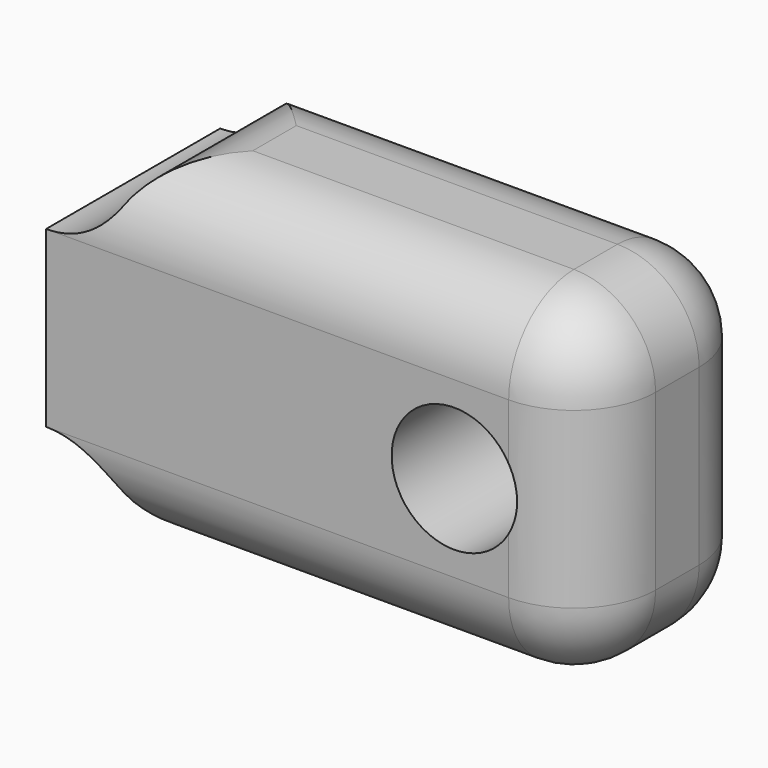
from build123d import *

# Parameters (mm, degrees)
F0_R         = 1.15
F1_DEPTH     = 4
F2_R         = 1.5
F3_DEPTH     = 5
F4_T1_DEPTH  = 9.4903810568
F4_T3_DEPTH  = 1
F4_T5_DEPTH  = 10.75
F4_T7_DEPTH  = 3.2
F4_S11_W     = 1.5
F4_S11_H     = 1.5
F4_T12_DEPTH = 1.5
F4_S17_W     = 1.5
F4_S17_H     = 1.5
F4_T18_DEPTH = 1.5
F4_S23_W     = 1.5
F4_S23_H     = 1.5
F4_T24_DEPTH = 1.5
F4_S29_W     = 1.5
F4_S29_H     = 1.5
F4_T30_DEPTH = 1.5


# Not quite as in the source:
# - a fillet or chamfer that OpenCascade refuses, or shapes differently, is made with other operations: its cross-section is extruded or revolved along the edge and cut away or added


with BuildPart() as f1:
    # F0 (on Front) → F1 (new body)
    with BuildSketch(Plane.XZ):
        with BuildLine():
            Line((5, 3.1), (-3.5, 3.1))
            ThreePointArc((-3.5, 3.1), (-3.9393398282, 2.0393398282), (-5, 1.6))
            Line((-5, 1.6), (-5, -1.6))
            ThreePointArc((-5, -1.6), (-3.9393398282, -2.0393398282), (-3.5, -3.1))
            Line((-3.5, -3.1), (5, -3.1))
            Line((5, -3.1), (5, 3.1))
        make_face()
        with Locations((2.5, 0)):
            Circle(F0_R, mode=Mode.SUBTRACT)
    extrude(amount=F1_DEPTH)

    # F2 (on face) → F3 (cut)
    with BuildSketch(Plane(origin=(-5, 0, 0), x_dir=(0, -1, 0), z_dir=(-1, 0, 0))):
        with Locations((1.9687709864, 0)):
            Circle(F2_R)
    extrude(amount=-F3_DEPTH, mode=Mode.SUBTRACT)

    # F4: fillet of radius 1.5 on 10 edges, made by hand

    # F4_s2 → F4_t1 (cut)
    with BuildSketch(Plane.XZ.offset(-2.7451905284)):
        with BuildLine():
            ThreePointArc((-2.4019237886, 3.1), (-3.1519237886, 2.8990381057), (-3.7009618943, 2.35))
            ThreePointArc((-3.7009618943, 2.35), (-3.5511112606, 2.7117714323), (-3.5, 3.1))
            Line((-3.5, 3.1), (-2.4019237886, 3.1))
        make_face()
        with BuildLine():
            ThreePointArc((-2.4019237886, -3.1), (-3.1519237886, -2.8990381057), (-3.7009618943, -2.35))
            ThreePointArc((-3.7009618943, -2.35), (-3.5511112606, -2.7117714323), (-3.5, -3.1))
            Line((-3.5, -3.1), (-2.4019237886, -3.1))
        make_face()
    extrude(amount=F4_T1_DEPTH, mode=Mode.SUBTRACT)

    # F4_s4 → F4_t3 (cut)
    with BuildSketch(Plane.XZ.offset(1.5)):
        with BuildLine():
            ThreePointArc((3.5, 3.1), (4.5606601718, 2.6606601718), (5, 1.6))
            Line((5, 1.6), (5, 3.1))
            Line((5, 3.1), (3.5, 3.1))
        make_face()
        with BuildLine():
            ThreePointArc((5, -1.6), (4.5606601718, -2.6606601718), (3.5, -3.1))
            Line((3.5, -3.1), (5, -3.1))
            Line((5, -3.1), (5, -1.6))
        make_face()
    extrude(amount=F4_T3_DEPTH, mode=Mode.SUBTRACT)

    # F4_s6 → F4_t5 (cut)
    with BuildSketch(Plane.YZ.offset(-7.25)):
        with BuildLine():
            ThreePointArc((-2.5, 3.1), (-3.5606601718, 2.6606601718), (-4, 1.6))
            Line((-4, 1.6), (-4, 3.1))
            Line((-4, 3.1), (-2.5, 3.1))
        make_face()
        with BuildLine():
            ThreePointArc((-1.5, 3.1), (-0.4393398282, 2.6606601718), (0, 1.6))
            Line((0, 1.6), (0, 3.1))
            Line((0, 3.1), (-1.5, 3.1))
        make_face()
        with BuildLine():
            ThreePointArc((0, -1.6), (-0.4393398282, -2.6606601718), (-1.5, -3.1))
            Line((-1.5, -3.1), (0, -3.1))
            Line((0, -3.1), (0, -1.6))
        make_face()
        with BuildLine():
            ThreePointArc((-4, -1.6), (-3.5606601718, -2.6606601718), (-2.5, -3.1))
            Line((-2.5, -3.1), (-4, -3.1))
            Line((-4, -3.1), (-4, -1.6))
        make_face()
    extrude(amount=F4_T5_DEPTH, mode=Mode.SUBTRACT)

    # F4_s8 → F4_t7 (cut)
    with BuildSketch(Plane.XY.offset(-1.6)):
        with BuildLine():
            ThreePointArc((5, -1.5), (4.5606601718, -0.4393398282), (3.5, 0))
            Line((3.5, 0), (5, 0))
            Line((5, 0), (5, -1.5))
        make_face()
        with BuildLine():
            ThreePointArc((5, -2.5), (4.5606601718, -3.5606601718), (3.5, -4))
            Line((3.5, -4), (5, -4))
            Line((5, -4), (5, -2.5))
        make_face()
    extrude(amount=F4_T7_DEPTH, mode=Mode.SUBTRACT)


with BuildPart() as f4_tool10:
    # F4_s11 → F4_t12 (new body)
    with BuildSketch(Plane.XY.offset(1.6)):
        with Locations((4.25, -0.75)):
            Rectangle(F4_S11_W, F4_S11_H)
    extrude(amount=F4_T12_DEPTH)

    # F4_s13 → F4_t14 (revolve, cut)
    with BuildSketch(Plane(origin=(3.5, -1.5, 1.6), x_dir=(-0.7071067812, -0.7071067812, 0), z_dir=(-0.7071067812, 0.7071067812, 0))):
        with BuildLine():
            ThreePointArc((0, -1.5), (1.5, 0), (0, 1.5))
            Line((0, 1.5), (0, -1.5))
        make_face()
    revolve(axis=Axis((3.5, -1.5, 1.6), (0, 0, 1)), mode=Mode.SUBTRACT)


with BuildPart() as f1_1:
    add(f1.part)

    # F4_t9: cut F4_tool10
    add(f4_tool10.part, mode=Mode.SUBTRACT)


with BuildPart() as f4_tool16:
    # F4_s17 → F4_t18 (new body)
    with BuildSketch(Plane.XY.offset(1.6)):
        with Locations((4.25, -3.25)):
            Rectangle(F4_S17_W, F4_S17_H)
    extrude(amount=F4_T18_DEPTH)

    # F4_s19 → F4_t20 (revolve, cut)
    with BuildSketch(Plane(origin=(3.5, -2.5, 1.6), x_dir=(-0.7071067812, 0.7071067812, 0), z_dir=(0.7071067812, 0.7071067812, 0))):
        with BuildLine():
            ThreePointArc((0, -1.5), (1.5, 0), (0, 1.5))
            Line((0, 1.5), (0, -1.5))
        make_face()
    revolve(axis=Axis((3.5, -2.5, 1.6), (0, 0, 1)), mode=Mode.SUBTRACT)


with BuildPart() as f1_2:
    add(f1_1.part)

    # F4_t15: cut F4_tool16
    add(f4_tool16.part, mode=Mode.SUBTRACT)


with BuildPart() as f4_tool22:
    # F4_s23 → F4_t24 (new body)
    with BuildSketch(Plane.YZ.offset(3.5)):
        with Locations((-0.75, -2.35)):
            Rectangle(F4_S23_W, F4_S23_H)
    extrude(amount=F4_T24_DEPTH)

    # F4_s25 → F4_t26 (revolve, cut)
    with BuildSketch(Plane(origin=(3.5, -1.5, -1.6), x_dir=(0, -0.7071067812, 0.7071067812), z_dir=(0, 0.7071067812, 0.7071067812))):
        with BuildLine():
            ThreePointArc((0, -1.5), (1.5, 0), (0, 1.5))
            Line((0, 1.5), (0, -1.5))
        make_face()
    revolve(axis=Axis((3.5, -1.5, -1.6), (1, 0, 0)), mode=Mode.SUBTRACT)


with BuildPart() as f1_3:
    add(f1_2.part)

    # F4_t21: cut F4_tool22
    add(f4_tool22.part, mode=Mode.SUBTRACT)


with BuildPart() as f4_tool28:
    # F4_s29 → F4_t30 (new body)
    with BuildSketch(Plane.YZ.offset(3.5)):
        with Locations((-3.25, -2.35)):
            Rectangle(F4_S29_W, F4_S29_H)
    extrude(amount=F4_T30_DEPTH)

    # F4_s31 → F4_t32 (revolve, cut)
    with BuildSketch(Plane(origin=(3.5, -2.5, -1.6), x_dir=(0, 0.7071067812, 0.7071067812), z_dir=(0, 0.7071067812, -0.7071067812))):
        with BuildLine():
            ThreePointArc((0, -1.5), (1.5, 0), (0, 1.5))
            Line((0, 1.5), (0, -1.5))
        make_face()
    revolve(axis=Axis((3.5, -2.5, -1.6), (1, 0, 0)), mode=Mode.SUBTRACT)


with BuildPart() as f1_4:
    add(f1_3.part)

    # F4_t27: cut F4_tool28
    add(f4_tool28.part, mode=Mode.SUBTRACT)


solid = f1_4.part
